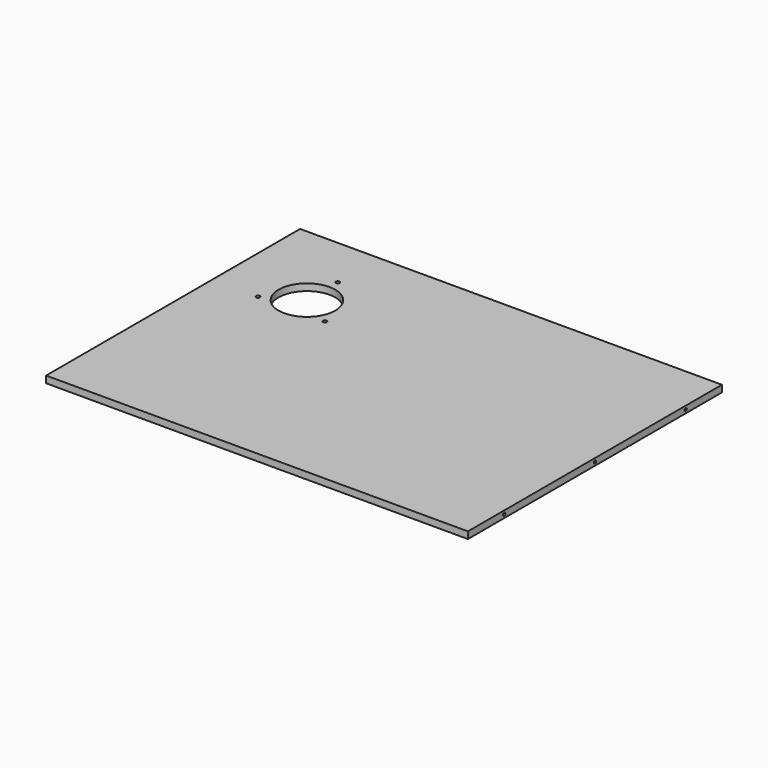
from build123d import *

# Parameters (mm, degrees)
F0_W           = 372
F0_H           = 280
F1_DEPTH       = 6
F2_R           = 25
F3_DEPTH       = 6
F5_D           = 3.4
F9_D           = 2.5
F9_DEPTH       = 16.5
F9_TIP         = 0.7510757738
F9_ON_F8_D     = 2.5
F9_ON_F8_DEPTH = 16.5
F9_ON_F8_TIP   = 0.7510757738
F9_ON_F7_D     = 2.5
F9_ON_F7_DEPTH = 16.5
F9_ON_F7_TIP   = 0.7510757738
F10_D          = 2.5
F10_DEPTH      = 16.5
F10_TIP        = 0.7510757738


# Not quite as in the source:
# - a feature names something its author has since deleted; it is built from what else it names


with BuildPart() as f1:
    # F0 (on Top) → F1 (new body)
    with BuildSketch(Plane.XY):
        Rectangle(F0_W, F0_H)
    extrude(amount=F1_DEPTH)


with BuildPart() as f3:
    # F2 (on face) → F3 (new body)
    with BuildSketch(Plane.XY.offset(6)):
        with Locations((-116, 60)):
            Circle(F2_R)
    extrude(amount=-F3_DEPTH)


with BuildPart() as f1_1:
    add(f1.part)

    # F4: cut F3
    add(f3.part, mode=Mode.SUBTRACT)

    # F5 (through all)
    with Locations(Plane.XY.offset(6)):
        with Locations((-116, 94), (-145.4448637287, 43), (-86.5551362713, 43)):
            Hole(F5_D / 2)

    # F9
    with Locations(Plane.YZ.offset(186)):
        with Locations((-100, 3), (0, 3), (100, 3)):
            Hole(F9_D / 2, depth=F9_DEPTH)
            with Locations((0, 0, -(F9_DEPTH + F9_TIP / 2))):  # 118° drill point
                Cone(0, F9_D / 2, F9_TIP, mode=Mode.SUBTRACT)

    # F9 on F8
    with Locations(Plane(origin=(0, 140, 0), x_dir=(-1, 0, 0), z_dir=(0, 1, 0))):
        with Locations((-150, 3), (-50, 3), (50, 3)):
            Hole(F9_ON_F8_D / 2, depth=F9_ON_F8_DEPTH)
            with Locations((0, 0, -(F9_ON_F8_DEPTH + F9_ON_F8_TIP / 2))):  # 118° drill point
                Cone(0, F9_ON_F8_D / 2, F9_ON_F8_TIP, mode=Mode.SUBTRACT)

    # F9 on F7
    with Locations(Plane(origin=(-186, 0, 0), x_dir=(0, -1, 0), z_dir=(-1, 0, 0))):
        with Locations((-100, 3), (0, 3), (100, 3)):
            Hole(F9_ON_F7_D / 2, depth=F9_ON_F7_DEPTH)
            with Locations((0, 0, -(F9_ON_F7_DEPTH + F9_ON_F7_TIP / 2))):  # 118° drill point
                Cone(0, F9_ON_F7_D / 2, F9_ON_F7_TIP, mode=Mode.SUBTRACT)

    # F10
    with Locations(Plane(origin=(0, 140, 0), x_dir=(-1, 0, 0), z_dir=(0, 1, 0))):
        with Locations((150, 3)):
            Hole(F10_D / 2, depth=F10_DEPTH)
            with Locations((0, 0, -(F10_DEPTH + F10_TIP / 2))):  # 118° drill point
                Cone(0, F10_D / 2, F10_TIP, mode=Mode.SUBTRACT)


solid = f1_1.part
